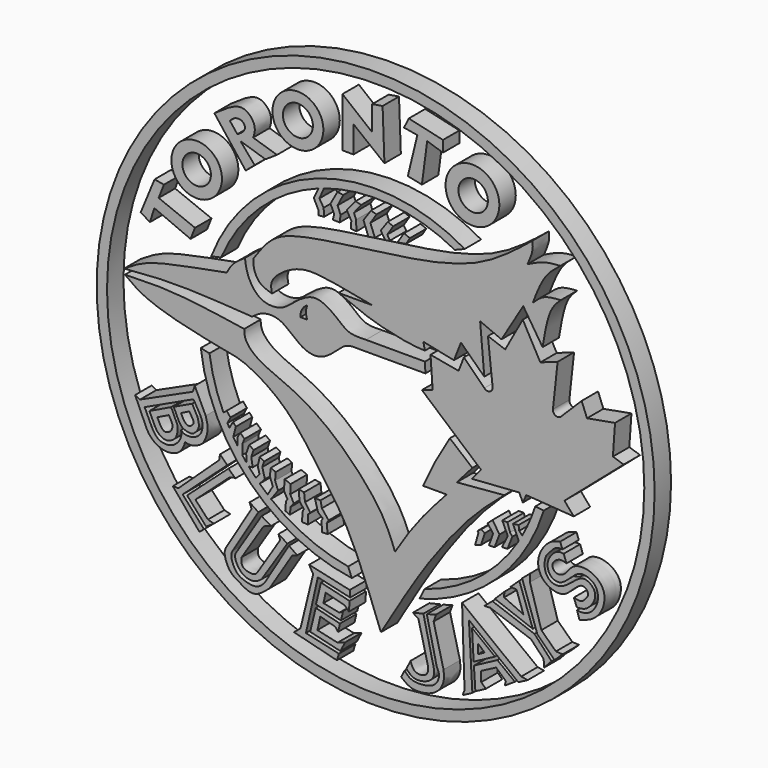
from build123d import *

# Parameters (mm, degrees)
F0_R     = 86.3413531424
F0_R_2   = 83.1380480695
F1_DEPTH = 6.35
F0_R_3   = 7.8789103403
F0_R_4   = 4.6380734479
F0_R_5   = 8.3244064096
F0_R_6   = 4.5488464078
F0_R_7   = 7.8253393062
F0_R_8   = 4.4151925566


with BuildPart() as f1:
    # F0 (on Front) → F1 (new body)
    with BuildSketch(Plane.XZ):
        with Locations((103.031180799, 95.9219709039)):
            Circle(F0_R)
        with Locations((103.031180799, 95.9219709039)):
            Circle(F0_R_2, mode=Mode.SUBTRACT)
    extrude(amount=F1_DEPTH)


with BuildPart() as f1b:
    # F0 (on Front) → F1, piece 2 (new body)
    with BuildSketch(Plane.XZ):
        with BuildLine():
            ThreePointArc((147.3083680993, 68.8155244448), (134.8042261554, 54.8646652976), (118.1625116195, 46.2604004246))
            Line((118.1625116195, 46.2604004246), (116.5973385643, 43.1300521934))
            ThreePointArc((116.5973385643, 43.1300521934), (140.56012864, 56.3921670644), (155.0479381108, 79.6344211676))
            Line((155.0479381108, 79.6344211676), (152.4171286424, 79.9139444647))
            ThreePointArc((152.4171286424, 79.9139444647), (150.6252567937, 75.1847414583), (148.3817446246, 70.6523227945))
            ThreePointArc((148.3817446246, 70.6523227945), (147.8544660424, 69.7284248505), (147.3083680993, 68.8155244448))
        make_face()
        with BuildLine():
            Line((145.5425322056, 72.9509443045), (147.3083680993, 68.8155244448))
            ThreePointArc((147.3083680993, 68.8155244448), (147.8544660424, 69.7284248505), (148.3817446246, 70.6523227945))
            Line((148.3817446246, 70.6523227945), (147.4613398314, 71.6612488031))
            Line((147.4613398314, 71.6612488031), (147.2726166248, 73.1711387634))
            Line((147.2726166248, 73.1711387634), (145.5425322056, 72.9509443045))
        make_face()
    extrude(amount=F1_DEPTH)


with BuildPart() as f1c:
    # F0 (on Front) → F1, piece 3 (new body)
    with BuildSketch(Plane.XZ):
        with BuildLine():
            Line((51.6026031998, 88.8275955975), (48.9147157589, 89.4077150596))
            ThreePointArc((48.9147157589, 89.4077150596), (64.1807826745, 57.6901270664), (95.6492936354, 41.9170168761))
            Line((95.6492936354, 41.9170168761), (94.5090451372, 44.7106249088))
            ThreePointArc((94.5090451372, 44.7106249088), (81.9000965732, 48.501447559), (70.6502899912, 55.3423372762))
            ThreePointArc((70.6502899912, 55.3423372762), (70.115809711, 55.7746534218), (69.5871006289, 56.2140087749))
            ThreePointArc((69.5871006289, 56.2140087749), (68.3513199524, 57.2886173538), (67.1500481163, 58.4016687693))
            ThreePointArc((67.1500481163, 58.4016687693), (66.5511264504, 58.983719868), (65.9616453548, 59.5753301125))
            ThreePointArc((65.9616453548, 59.5753301125), (64.8429965328, 60.752504924), (63.7617125025, 61.9640908968))
            ThreePointArc((63.7617125025, 61.9640908968), (63.43044974, 62.350988576), (63.1029986811, 62.7411175751))
            ThreePointArc((63.1029986811, 62.7411175751), (62.4252381027, 63.5740780419), (61.7648512125, 64.4208789018))
            ThreePointArc((61.7648512125, 64.4208789018), (61.0137454914, 65.429941043), (60.2873081661, 66.4569050257))
            ThreePointArc((60.2873081661, 66.4569050257), (59.6233759404, 67.4440631116), (58.9822375149, 68.4461751843))
            ThreePointArc((58.9822375149, 68.4461751843), (58.3639510652, 69.4631851651), (57.7691413004, 70.4941016402))
            ThreePointArc((57.7691413004, 70.4941016402), (57.4587222425, 71.0547278725), (57.155246887, 71.6191430321))
            ThreePointArc((57.155246887, 71.6191430321), (56.5262459763, 72.8455805448), (55.9300250893, 74.0882839575))
            ThreePointArc((55.9300250893, 74.0882839575), (53.2181412071, 81.296997691), (51.6026031998, 88.8275955975))
        make_face()
        with BuildLine():
            Line((56.9120161235, 74.9070867896), (55.9300250893, 74.0882839575))
            ThreePointArc((55.9300250893, 74.0882839575), (56.5262459763, 72.8455805448), (57.155246887, 71.6191430321))
            Line((57.155246887, 71.6191430321), (58.1148564816, 73.4815001488))
            Line((58.1148564816, 73.4815001488), (56.9120161235, 74.9070867896))
        make_face()
        with BuildLine():
            Line((58.8709115982, 72.4884793162), (57.7691413004, 70.4941016402))
            ThreePointArc((57.7691413004, 70.4941016402), (58.3639510652, 69.4631851651), (58.9822375149, 68.4461751843))
            Line((58.9822375149, 68.4461751843), (59.7831308842, 71.5290755033))
            Line((59.7831308842, 71.5290755033), (58.8709115982, 72.4884793162))
        make_face()
        with BuildLine():
            Line((60.2873081661, 68.8241523461), (60.2873081661, 66.4569050257))
            ThreePointArc((60.2873081661, 66.4569050257), (61.0137454914, 65.429941043), (61.7648512125, 64.4208789018))
            Line((61.7648512125, 64.4208789018), (61.7648512125, 67.4240812659))
            Line((61.7648512125, 67.4240812659), (62.4568797648, 69.0440535545))
            Line((62.4568797648, 69.0440535545), (61.1357353628, 70.2865645289))
            Line((61.1357353628, 70.2865645289), (60.2873081661, 68.8241523461))
        make_face()
        with BuildLine():
            ThreePointArc((63.1029986811, 62.7411175751), (63.43044974, 62.350988576), (63.7617125025, 61.9640908968))
            Line((63.7617125025, 61.9640908968), (65.0048106909, 62.123760581))
            Line((65.0048106909, 62.123760581), (64.5329728723, 64.7660568357))
            Line((64.5329728723, 64.7660568357), (65.2721822262, 66.920787096))
            Line((65.2721822262, 66.920787096), (63.9195814729, 67.9273754358))
            Line((63.9195814729, 67.9273754358), (62.96017766, 65.2536228299))
            Line((62.96017766, 65.2536228299), (63.1029986811, 62.7411175751))
        make_face()
        with BuildLine():
            ThreePointArc((65.9616453548, 59.5753301125), (66.5511264504, 58.983719868), (67.1500481163, 58.4016687693))
            Line((67.1500481163, 58.4016687693), (68.748511374, 60.1065568626))
            Line((68.748511374, 60.1065568626), (67.9659470916, 63.1837621331))
            Line((67.9659470916, 63.1837621331), (68.4965029359, 64.8682713509))
            Line((68.4965029359, 64.8682713509), (67.1833828092, 65.7171532512))
            Line((67.1833828092, 65.7171532512), (66.5334537625, 63.0643889308))
            Line((66.5334537625, 63.0643889308), (67.0905336738, 60.9023831785))
            Line((67.0905336738, 60.9023831785), (65.9616453548, 59.5753301125))
        make_face()
        with BuildLine():
            ThreePointArc((69.5871006289, 56.2140087749), (70.115809711, 55.7746534218), (70.6502899912, 55.3423372762))
            Line((70.6502899912, 55.3423372762), (72.8397592902, 58.3484321833))
            Line((72.8397592902, 58.3484321833), (71.9113647938, 60.7402287424))
            Line((71.9113647938, 60.7402287424), (72.1001923084, 63.1477609277))
            Line((72.1001923084, 63.1477609277), (70.5895796418, 63.8243928552))
            Line((70.5895796418, 63.8243928552), (70.2748671174, 61.4325925708))
            Line((70.2748671174, 61.4325925708), (71.2347403169, 58.9463822544))
            Line((71.2347403169, 58.9463822544), (69.5871006289, 56.2140087749))
        make_face()
    extrude(amount=F1_DEPTH)


with BuildPart() as f1d:
    # F0 (on Front) → F1, piece 4 (new body)
    with BuildSketch(Plane.XZ):
        with BuildLine():
            ThreePointArc((130.5909766711, 142.9483993153), (84.998217789, 147.3596959967), (52.1404570115, 115.4453299904))
            Line((52.1404570115, 115.4453299904), (55.2052152042, 116.1186481005))
            ThreePointArc((55.2052152042, 116.1186481005), (67.2921720529, 133.5776744388), (85.3582697834, 144.7368966039))
            ThreePointArc((85.3582697834, 144.7368966039), (86.1877646377, 145.0292828532), (87.0220936823, 145.3075749253))
            ThreePointArc((87.0220936823, 145.3075749253), (107.6444471834, 147.632187768), (127.5296217117, 141.6937432938))
            Line((127.5296217117, 141.6937432938), (130.5909766711, 142.9483993153))
        make_face()
        with BuildLine():
            ThreePointArc((87.0220936823, 145.3075749253), (86.1877646377, 145.0292828532), (85.3582697834, 144.7368966039))
            Line((85.3582697834, 144.7368966039), (83.8721096516, 141.6685283184))
            Line((83.8721096516, 141.6685283184), (85.278019309, 138.902798295))
            Line((85.278019309, 138.902798295), (85.278019309, 137.4046951532))
            Line((85.278019309, 137.4046951532), (87.0757475495, 137.5429779291))
            Line((87.0757475495, 137.5429779291), (86.9374573231, 139.986038208))
            Line((86.9374573231, 139.986038208), (85.6237336993, 142.1064287424))
            Line((85.6237336993, 142.1064287424), (87.0220936823, 145.3075749253))
        make_face()
    extrude(amount=F1_DEPTH)


with BuildPart() as f1e:
    # F0 (on Front) → F1, piece 5 (new body)
    with BuildSketch(Plane.XZ):
        with BuildLine():
            add(Edge.make_bspline(
                [(65.1605650783, 119.0443858504), (66.8778376252, 121.5129392999), (70.4109060542, 126.5916720109), (79.9235957481, 130.7139890188), (110.1374116444, 133.9828883244), (135.222430189, 138.8339439937), (146.3601247065, 147.8218221424), (151.5567153692, 152.0153582096)],
                knots=[0, 0, 0, 0, 0.1391278046, 0.2862376476, 0.5460671762, 0.7882054433, 1, 1, 1, 1], degree=3))
            add(Edge.make_bspline(
                [(65.1605650783, 119.0443858504), (65.1761761693, 118.1416763553), (65.2095890258, 116.209581882), (66.9509015853, 112.6183397292), (69.5998832246, 111.8216078708), (70.9610208869, 111.4122197032)],
                knots=[0, 0, 0, 0, 0.2989041205, 0.63975288, 1, 1, 1, 1], degree=3))
            add(Edge.make_bspline(
                [(70.9610208869, 111.4122197032), (70.7064543789, 112.6000383971), (70.0542774567, 115.6431250383), (78.5588548833, 121.5103784794), (86.7278880375, 121.319656762), (96.3330449421, 119.4304990241), (101.8915474415, 118.3372437954)],
                knots=[0, 0, 0, 0, 0.1632480059, 0.4182269808, 0.6633280629, 1, 1, 1, 1], degree=3))
            add(Edge.make_bspline(
                [(91.5042832494, 118.2865723968), (94.9667046467, 118.303462863), (98.4291260441, 118.3203533292), (101.8915474415, 118.3372437954)],
                knots=[0, 0, 0, 0, 10.3873877846, 10.3873877846, 10.3873877846, 10.3873877846], degree=3))
            add(Edge.make_bspline(
                [(91.5042832494, 118.2865723968), (95.4103000455, 116.6689675882), (102.9409801099, 113.550275345), (114.0365493527, 111.4182928611), (117.1070508324, 111.2911466343), (118.2578355074, 111.243493855)],
                knots=[0, 0, 0, 0, 0.4025367258, 0.7760784079, 1, 1, 1, 1], degree=3))
            Line((118.2578355074, 111.243493855), (117.8089082241, 113.522939384))
            Line((117.8089082241, 113.522939384), (127.2610574961, 111.5468814969))
            Line((127.2610574961, 111.5468814969), (129.4347345829, 117.079846561))
            Line((129.4347345829, 117.079846561), (136.6473585367, 110.1306974888))
            Line((136.6473585367, 110.1306974888), (135.3629082441, 124.8194202781))
            Line((135.3629082441, 124.8194202781), (141.9620066881, 122.0207512379))
            Line((141.9620066881, 122.0207512379), (148.6962139606, 133.2910507917))
            Line((148.6962139606, 133.2910507917), (154.6910554171, 124.0390092134))
            add(Edge.make_bspline(
                [(160.315155983, 138.6734396219), (159.2455875755, 137.6606965238), (156.5295767546, 135.0889851736), (155.384935522, 128.2094032809), (154.6910554171, 124.0390092134)],
                knots=[0, 0, 0, 0, 0.393801232, 1, 1, 1, 1], degree=3))
            add(Edge.make_bspline(
                [(151.6671776772, 135.1648271084), (152.7209926622, 136.1815330098), (154.935600551, 138.3181556068), (158.4651387096, 138.551258231), (160.315155983, 138.6734396219)],
                knots=[0, 0, 0, 0, 0.4758472099, 1, 1, 1, 1], degree=3))
            add(Edge.make_bspline(
                [(160.1669043303, 147.9638516903), (158.5547438369, 146.6889334698), (154.9894110066, 143.8694202723), (152.843020417, 138.2456560751), (151.6671776772, 135.1648271084)],
                knots=[0, 0, 0, 0, 0.4521767168, 1, 1, 1, 1], degree=3))
            add(Edge.make_bspline(
                [(150.0364094973, 145.1470702887), (151.760692317, 145.9999334812), (155.1077875128, 147.6554706482), (158.5149626664, 147.8631567449), (160.1669043303, 147.9638516903)],
                knots=[0, 0, 0, 0, 0.5151579859, 1, 1, 1, 1], degree=3))
            add(Edge.make_bspline(
                [(151.5567153692, 152.0153582096), (151.6401552323, 151.1871213753), (151.8331461293, 149.2714642344), (150.6870113993, 146.6405215258), (150.0364094973, 145.1470702887)],
                knots=[0, 0, 0, 0, 0.432351289, 1, 1, 1, 1], degree=3))
        make_face()
    extrude(amount=F1_DEPTH)


with BuildPart() as f1f:
    # F0 (on Front) → F1, piece 6 (new body)
    with BuildSketch(Plane.XZ):
        with BuildLine():
            add(Edge.make_bspline(
                [(25.1967553049, 103.3449247479), (27.3040968371, 104.7393627023), (32.4641344694, 108.1537842428), (50.5762950972, 111.2823313326), (55.2229375422, 112.2109965294), (56.9541603327, 112.5569939613)],
                knots=[0, 0, 0, 0, 0.3022241239, 0.7400261557, 1, 1, 1, 1], degree=3))
            add(Edge.make_bspline(
                [(25.1967553049, 103.3449247479), (29.9715334206, 103.7590919436), (40.7871203818, 104.6972426205), (56.1858731237, 103.685420688), (64.7865086794, 103.1202897429)],
                knots=[0, 0, 0, 0, 0.4414719361, 1, 1, 1, 1], degree=3))
            add(Edge.make_bspline(
                [(64.7865086794, 103.1202897429), (65.8668973717, 103.9080368704), (68.1814863805, 105.5956802675), (74.1229212632, 105.629850452), (79.4777048259, 99.5938625168), (85.4832150354, 98.1867823774), (90.0852174163, 101.3548826723), (93.694568367, 105.2928580339), (98.082420715, 105.0210518449), (99.9919539194, 105.0507986742), (100.8540317416, 105.0642281771)],
                knots=[0, 0, 0, 0, 0.1136037838, 0.2433809899, 0.4013829827, 0.5347427751, 0.6644027588, 0.7926653345, 0.9063966961, 1, 1, 1, 1], degree=3))
            Line((100.8540317416, 105.0642281771), (118.4250637889, 105.0808951259))
            Line((118.4250637889, 105.0808951259), (118.2891801, 108.2712113857))
            Line((118.2891801, 108.2712113857), (100.034929812, 108.2712113857))
            add(Edge.make_bspline(
                [(62.5645443797, 118.3710470796), (62.7810828536, 116.8203199403), (63.2439830099, 113.5052885639), (67.1459023608, 107.817655531), (73.9886371488, 107.8306557792), (77.4019191042, 111.1699255534), (81.1499566889, 113.7985632868), (85.4234713853, 115.2807346354), (91.3316282439, 111.2904547181), (94.4912731866, 108.103824159), (98.1342859466, 108.2138226391), (100.034929812, 108.2712113857)],
                knots=[0, 0, 0, 0, 0.1079264135, 0.2307172152, 0.3501145928, 0.455522384, 0.5593277087, 0.6585426343, 0.7849741393, 0.887816044, 1, 1, 1, 1], degree=3))
            add(Edge.make_bspline(
                [(62.5645443797, 118.3710470796), (62.1619489758, 118.1183126282), (61.1729889871, 117.4974802547), (58.4413848848, 115.3726745542), (57.4458065929, 113.4878008334), (56.9541603327, 112.5569939613)],
                knots=[0, 0, 0, 0, 0.2579038412, 0.6335307789, 1, 1, 1, 1], degree=3))
        make_face()
        with BuildLine():
            ThreePointArc((79.7450765967, 107.8225299716), (80.2463337926, 110.1185380343), (81.8977057934, 111.7906272411))
            ThreePointArc((81.8977057934, 111.7906272411), (81.4659620101, 109.8248859653), (81.8458348513, 107.8484654427))
            Line((81.8458348513, 107.8484654427), (79.7450765967, 107.8225299716))
        make_face(mode=Mode.SUBTRACT)
    extrude(amount=F1_DEPTH)


with BuildPart() as f1g:
    # F0 (on Front) → F1, piece 7 (new body)
    with BuildSketch(Plane.XZ):
        with BuildLine():
            Line((153.9957672358, 119.6609884501), (148.5578864813, 129.5398026705))
            Line((148.5578864813, 129.5398026705), (143.1200057268, 119.6609884501))
            Line((143.1200057268, 119.6609884501), (137.7727538347, 121.5642467141))
            Line((137.7727538347, 121.5642467141), (139.2228603363, 108.1508100033))
            ThreePointArc((139.2228603363, 108.1508100033), (138.3571175254, 106.656984618), (136.6722881794, 107.0343106985))
            Line((136.6722881794, 107.0343106985), (130.3365975618, 113.3399754763))
            Line((130.3365975618, 113.3399754763), (128.6851167679, 109.1362014413))
            Line((128.6851167679, 109.1362014413), (120.0073137879, 110.6976047158))
            Line((120.0073137879, 110.6976047158), (120.6679046154, 101.2991517782))
            Line((120.6679046154, 101.2991517782), (117.3349097371, 100.2181842923))
            Line((117.3349097371, 100.2181842923), (135.6661170721, 84.4167545438))
            Line((135.6661170721, 84.4167545438), (132.773819657, 81.0614060446))
            Line((132.773819657, 81.0614060446), (147.4750339985, 82.0971429348))
            Line((147.4750339985, 82.0971429348), (148.5578864813, 79.6925723553))
            Line((148.5578864813, 79.6925723553), (149.6407389641, 82.0971429348))
            Line((149.6407389641, 82.0971429348), (164.3419533056, 81.0614060446))
            Line((164.3419533056, 81.0614060446), (161.4496558905, 84.4167545438))
            Line((161.4496558905, 84.4167545438), (179.7808632255, 100.2181842923))
            Line((179.7808632255, 100.2181842923), (176.4478683472, 101.2991517782))
            Line((176.4478683472, 101.2991517782), (177.1084591746, 110.6976047158))
            Line((177.1084591746, 110.6976047158), (168.4306561947, 109.1362014413))
            Line((168.4306561947, 109.1362014413), (166.7791754007, 113.3399754763))
            Line((166.7791754007, 113.3399754763), (160.4434847832, 107.0343106985))
            ThreePointArc((160.4434847832, 107.0343106985), (158.7586554371, 106.656984618), (157.8929126263, 108.1508100033))
            Line((157.8929126263, 108.1508100033), (159.3430191278, 121.5642467141))
            Line((159.3430191278, 121.5642467141), (153.9957672358, 119.6609884501))
        make_face()
    extrude(amount=F1_DEPTH)


with BuildPart() as f1h:
    # F0 (on Front) → F1, piece 8 (new body)
    with BuildSketch(Plane.XZ):
        with BuildLine():
            add(Edge.make_bspline(
                [(25.4391785711, 101.7691716552), (30.0819421715, 101.9373475003), (40.4646043806, 102.313440953), (54.5665174618, 100.1663488978), (62.3625479639, 98.9793613553)],
                knots=[0, 0, 0, 0, 0.4471650437, 1, 1, 1, 1], degree=3))
            add(Edge.make_bspline(
                [(25.4391785711, 101.7691716552), (27.4951677939, 100.2010333845), (32.6963862517, 96.2339747892), (53.7919926338, 91.5360298149), (62.6667020346, 90.4660345952), (76.1675062641, 81.8773948587), (85.1809430093, 68.5570252624), (94.9490355887, 55.8282536231), (101.1341707007, 39.4515366233), (104.6594902873, 30.1173571497)],
                knots=[0, 0, 0, 0, 0.1078526072, 0.2728443151, 0.3840716275, 0.52293785, 0.667189915, 0.8103094128, 1, 1, 1, 1], degree=3))
            add(Edge.make_bspline(
                [(142.8586542606, 79.8605903983), (139.8099959288, 77.2901032161), (132.7752691758, 71.3587481803), (118.9267540138, 54.1605827862), (109.6282733945, 38.4907618667), (104.6594902873, 30.1173571497)],
                knots=[0, 0, 0, 0, 0.2626080184, 0.6059634932, 1, 1, 1, 1], degree=3))
            Line((142.8586542606, 79.8605903983), (128.1391531229, 78.5893574357))
            Line((128.1391531229, 78.5893574357), (132.9556107521, 84.0778797865))
            Line((132.9556107521, 84.0778797865), (125.9915083647, 89.889511466))
            add(Edge.make_bspline(
                [(125.9915083647, 89.889511466), (124.1906776032, 86.884529911), (120.831371918, 81.2789772755), (118.6989388734, 76.4671217587), (117.7096441388, 74.2347687483)],
                knots=[0, 0, 0, 0, 0.5360723109, 1, 1, 1, 1], degree=3))
            Line((117.7096441388, 74.2347687483), (124.9815225601, 74.2347687483))
            add(Edge.make_bspline(
                [(109.0237796307, 53.4291043878), (111.0607083235, 56.6835559182), (115.3540422303, 63.5431220642), (121.6648260608, 70.5514636763), (124.9815225601, 74.2347687483)],
                knots=[0, 0, 0, 0, 0.4744398496, 1, 1, 1, 1], degree=3))
            add(Edge.make_bspline(
                [(62.3625479639, 98.9793613553), (62.3939304569, 98.0520448539), (62.470120325, 95.8007220626), (67.1036326561, 91.1212871301), (79.0408742875, 87.1555023958), (92.4624754667, 77.7456992381), (105.2124808885, 63.5789766808), (107.8826662406, 56.468004239), (109.0237796307, 53.4291043878)],
                knots=[0, 0, 0, 0, 0.0876826859, 0.212874492, 0.3948990845, 0.6080658661, 0.8325055271, 1, 1, 1, 1], degree=3))
        make_face()
    extrude(amount=F1_DEPTH)


with BuildPart() as f1i:
    # F0 (on Front) → F1, piece 9 (new body)
    with BuildSketch(Plane.XZ):
        Polygon((45.7493290305, 118.0791184306), (47.1274256706, 121.5687170625), (35.8816534281, 126.0549873114), (37.5066287816, 130.2057057619), (34.6122793853, 130.7036727667), (30.3303021938, 120.3440725803), (33.1689864397, 118.5628324747), (34.5361232758, 122.8588074446), align=None)
    extrude(amount=F1_DEPTH)


with BuildPart() as f1j:
    # F0 (on Front) → F1, piece 10 (new body)
    with BuildSketch(Plane.XZ):
        with BuildLine():
            add(Edge.make_bspline(
                [(53.1252250075, 154.7500044107), (55.2469486953, 156.2413880414), (58.8098820474, 158.7458142818), (62.4338563704, 159.3498216887), (65.3452902263, 156.7860195347), (65.8141525821, 153.9353043584), (65.3288470884, 152.6082080035), (65.105214715, 151.9966721535)],
                knots=[0, 0, 0, 0, 0.283267468, 0.4756807474, 0.6736240285, 0.84960353, 1, 1, 1, 1], degree=3))
            Line((53.1252250075, 154.7500044107), (62.8135204315, 142.2608792782))
            Line((62.8135204315, 142.2608792782), (65.5893757939, 144.6471214294))
            Line((65.5893757939, 144.6471214294), (61.1652935744, 149.7935447907))
            Line((61.1652935744, 149.7935447907), (68.9228177071, 147.3327279091))
            Line((68.9228177071, 147.3327279091), (72.4971592426, 149.693518877))
            Line((72.4971592426, 149.693518877), (65.105214715, 151.9966721535))
        make_face()
        with BuildLine():
            Line((60.2364838123, 151.348516345), (57.8906238079, 154.3007344007))
            add(Edge.make_bspline(
                [(57.8906238079, 154.3007344007), (58.4380867229, 154.7951363586), (59.5217921733, 155.7738073915), (61.9341600232, 155.7245852448), (62.9476560436, 153.6651432613), (61.6809151257, 152.170733141), (60.7159422125, 151.6214394989), (60.2364838123, 151.348516345)],
                knots=[0, 0, 0, 0, 0.2140840398, 0.4237803775, 0.6200878393, 0.8112360728, 1, 1, 1, 1], degree=3))
        make_face(mode=Mode.SUBTRACT)
    extrude(amount=F1_DEPTH)


with BuildPart() as f1k:
    # F0 (on Front) → F1, piece 11 (new body)
    with BuildSketch(Plane.XZ):
        with Locations((78.9697542787, 161.17811203)):
            Circle(F0_R_3)
        with Locations((78.9697542787, 161.17811203)):
            Circle(F0_R_4, mode=Mode.SUBTRACT)
    extrude(amount=F1_DEPTH)


with BuildPart() as f1l:
    # F0 (on Front) → F1, piece 12 (new body)
    with BuildSketch(Plane.XZ):
        Polygon((105.7477369905, 158.2026481628), (105.1767095923, 173.6358851194), (101.9640862942, 173.1107831001), (101.9640862942, 165.42981565), (92.7540138364, 172.8455275297), (92.7540138364, 157.5022041798), (96.1784869432, 157.5022041798), (96.1784869432, 165.7617539167), align=None)
    extrude(amount=F1_DEPTH)


with BuildPart() as f1m:
    # F0 (on Front) → F1, piece 13 (new body)
    with BuildSketch(Plane.XZ):
        Polygon((112.9893511534, 157.0811718702), (117.3376590014, 156.1619192362), (118.9757287502, 168.5630083084), (123.8637119532, 166.9919341803), (123.8637119532, 170.4729348421), (113.2804900408, 172.8813052177), (111.8034347892, 169.9022501707), (115.9320175648, 169.1992431879), align=None)
    extrude(amount=F1_DEPTH)


with BuildPart() as f1n:
    # F0 (on Front) → F1, piece 14 (new body)
    with BuildSketch(Plane.XZ):
        with Locations((132.9881995916, 158.4182977676)):
            Circle(F0_R_5)
        with Locations((133.2059800625, 158.3469808102)):
            Circle(F0_R_6, mode=Mode.SUBTRACT)
    extrude(amount=F1_DEPTH)


with BuildPart() as f1o:
    # F0 (on Front) → F1, piece 15 (new body)
    with BuildSketch(Plane.XZ):
        with BuildLine():
            Line((30.084611848, 69.2335367203), (28.5908672959, 69.9970424175))
            Line((28.5908672959, 69.9970424175), (32.2739779949, 61.7518611252))
            add(Edge.make_bspline(
                [(32.2739779949, 61.7518611252), (32.7749833614, 60.9635409459), (33.8725362138, 59.2365673057), (37.7843402929, 57.3661795763), (40.9000261821, 58.0772316706), (42.4748576233, 58.8884277898), (43.7190339293, 60.8511833229), (43.92516752, 61.788340814), (44.0159887075, 62.2012466192)],
                knots=[0, 0, 0, 0, 0.1805400151, 0.3955091539, 0.5798726097, 0.7192386574, 0.8762982857, 1, 1, 1, 1], degree=3))
            add(Edge.make_bspline(
                [(50.4372827709, 71.4342072606), (50.768796352, 70.2681071733), (51.4423387053, 67.8989197804), (50.0208490553, 63.9368372151), (48.3439726978, 62.6064898882), (45.6286973181, 61.7319686813), (44.5064816628, 62.0585193335), (44.0159887075, 62.2012466192)],
                knots=[0, 0, 0, 0, 0.2317101951, 0.4707699442, 0.6474136486, 0.8458931484, 1, 1, 1, 1], degree=3))
            Line((50.4372827709, 71.4342072606), (47.0445714891, 78.5238817334))
            Line((47.0445714891, 78.5238817334), (46.4649833739, 76.70263201))
            Line((46.4649833739, 76.70263201), (30.084611848, 69.2335367203))
        make_face()
        with BuildLine():
            Line((33.7571738878, 62.9248380445), (31.5462499857, 67.6518827677))
            Line((31.5462499857, 67.6518827677), (46.6555319726, 74.7187659144))
            Line((46.6555319726, 74.7187659144), (48.8234609365, 70.9855034947))
            add(Edge.make_bspline(
                [(48.8234609365, 70.9855034947), (49.0819708256, 70.3935862537), (49.6586394805, 69.0731720892), (49.237163999, 65.7047735608), (46.3921689965, 63.9972381576), (43.6765691296, 64.193013021), (43.0678826774, 64.8492305233), (42.8228862584, 65.1133581996)],
                knots=[0, 0, 0, 0, 0.1877571763, 0.4188376649, 0.6505028982, 0.8593273465, 1, 1, 1, 1], degree=3))
            add(Edge.make_bspline(
                [(42.8228862584, 65.1133581996), (42.8995880194, 64.5288190639), (43.0701928475, 63.2286507568), (41.5554270585, 60.7324634798), (38.9094693245, 59.408386698), (35.4556323147, 59.9614920092), (34.3283304255, 61.9283258929), (33.7571738878, 62.9248380445)],
                knots=[0, 0, 0, 0, 0.1629627988, 0.3624719943, 0.5673253374, 0.7807819142, 1, 1, 1, 1], degree=3))
        make_face(mode=Mode.SUBTRACT)
    extrude(amount=F1_DEPTH)


with BuildPart() as f1p:
    # F0 (on Front) → F1, piece 16 (new body)
    with BuildSketch(Plane.XZ):
        with BuildLine():
            Line((33.0113917589, 67.0752748847), (34.7925238311, 63.375480473))
            add(Edge.make_bspline(
                [(34.7925238311, 63.375480473), (35.0775184998, 62.8565718788), (35.6921398313, 61.7374902743), (38.0879074589, 60.4498929431), (40.1144582874, 61.3870935102), (41.5870528741, 62.6273809347), (41.9177078829, 65.8310003744), (41.5595239996, 66.4209627993), (41.4349101484, 66.626213491)],
                knots=[0, 0, 0, 0, 0.1617435236, 0.348817121, 0.5186377126, 0.6833715959, 0.8898434947, 1, 1, 1, 1], degree=3))
            Line((41.4349101484, 66.626213491), (39.7495812228, 70.3191322528))
            Line((39.7495812228, 70.3191322528), (33.0113917589, 67.0752748847))
        make_face()
        with BuildLine():
            add(Edge.make_bspline(
                [(39.0181578696, 67.9107233882), (39.3521406209, 67.3612992199), (39.9734686595, 66.3391726595), (40.3585117661, 64.9323679736), (39.4065180237, 63.2149036456), (37.5045449143, 62.7910345829), (36.4835226493, 64.0908443815), (35.8268386909, 65.4262056166), (35.4576520622, 66.176943481)],
                knots=[0, 0, 0, 0, 0.1723413883, 0.320616967, 0.4896060074, 0.6516265134, 0.8041450056, 1, 1, 1, 1], degree=3))
            Line((35.4576520622, 66.176943481), (39.0181578696, 67.9107233882))
        make_face(mode=Mode.SUBTRACT)
    extrude(amount=F1_DEPTH)


with BuildPart() as f1q:
    # F0 (on Front) → F1, piece 17 (new body)
    with BuildSketch(Plane.XZ):
        with BuildLine():
            Line((40.5272841454, 70.6554576755), (42.1947091818, 67.1063810587))
            add(Edge.make_bspline(
                [(42.1947091818, 67.1063810587), (42.5300203172, 66.6059812645), (43.2534498254, 65.5263750754), (45.9643010197, 64.9343952109), (47.0261507091, 65.6262016891), (48.7203927869, 67.4674823606), (48.1852515678, 69.3114875856), (47.9004643857, 70.2928155661)],
                knots=[0, 0, 0, 0, 0.1892913736, 0.4083937301, 0.5618475325, 0.7668275175, 1, 1, 1, 1], degree=3))
            Line((47.9004643857, 70.2928155661), (46.2758727372, 73.3677372336))
            Line((46.2758727372, 73.3677372336), (40.5272841454, 70.6554576755))
        make_face()
        with BuildLine():
            add(Edge.make_bspline(
                [(42.7959747612, 69.7186216712), (43.047642654, 69.1511576598), (43.5409352666, 68.0388751126), (44.9829181822, 66.4963706403), (46.8393950574, 67.849105025), (46.5990822652, 69.119399867), (45.7980453979, 70.2741922494), (45.3262329102, 70.9543675184)],
                knots=[0, 0, 0, 0, 0.2093713151, 0.4103873638, 0.6113362611, 0.7710761976, 1, 1, 1, 1], degree=3))
            Line((42.7959747612, 69.7186216712), (45.3262329102, 70.9543675184))
        make_face(mode=Mode.SUBTRACT)
    extrude(amount=F1_DEPTH)


with BuildPart() as f1r:
    # F0 (on Front) → F1, piece 18 (new body)
    with BuildSketch(Plane.XZ):
        Polygon((42.0019701123, 48.9689558744), (40.2475222945, 48.9689558744), (48.4948754311, 39.1794070601), (49.9138982921, 40.3748842845), (43.3076843619, 47.6965904236), (57.1298776725, 60.1680505258), (54.8735894263, 62.4050199986), (54.5935668051, 60.7121512294), align=None)
    extrude(amount=F1_DEPTH)


with BuildPart() as f1s:
    # F0 (on Front) → F1, piece 19 (new body)
    with BuildSketch(Plane.XZ):
        Polygon((59.1355338693, 57.3903694749), (59.5765225589, 57.3363490403), (57.5092588319, 59.385912458), (44.6798056364, 47.8761643171), (50.5935712321, 41.2843277287), (52.980992943, 42.9032854736), (51.1294156313, 43.4014163911), (47.2444631159, 47.572825104), (57.8899629671, 57.1232728319), align=None)
    extrude(amount=F1_DEPTH)


with BuildPart() as f1t:
    # F0 (on Front) → F1, piece 20 (new body)
    with BuildSketch(Plane.XZ):
        with BuildLine():
            Line((66.7242109776, 50.4824742675), (64.0202015638, 52.2900372744))
            Line((64.0202015638, 52.2900372744), (64.6236911416, 50.680808723))
            Line((64.6236911416, 50.680808723), (56.8242445588, 37.761926651))
            add(Edge.make_bspline(
                [(56.8242445588, 37.761926651), (56.5676145385, 37.2745883782), (55.9068287024, 36.0197615746), (57.5079599547, 31.3390733944), (60.8664515095, 29.4597501756), (65.4071147291, 26.6832553249), (68.507722817, 29.3797027929), (70.1521411538, 30.8097731322)],
                knots=[0, 0, 0, 0, 0.1342385427, 0.3456451728, 0.5458891784, 0.7591607385, 1, 1, 1, 1], degree=3))
            Line((70.1521411538, 30.8097731322), (77.2129967809, 42.0901700854))
            Line((77.2129967809, 42.0901700854), (78.7653923035, 42.636051774))
            Line((78.7653923035, 42.636051774), (76.2063041329, 44.4313026965))
            Line((76.2063041329, 44.4313026965), (68.6753094196, 31.8774543703))
            add(Edge.make_bspline(
                [(58.728441596, 37.323653698), (58.5230264271, 36.8687220199), (57.9958517355, 35.701191558), (59.6709627467, 31.6246690145), (62.6263598052, 30.2447432329), (66.4668279016, 29.5192915207), (67.9592674068, 31.1128821247), (68.6753094196, 31.8774543703)],
                knots=[0, 0, 0, 0, 0.1465737445, 0.3761648615, 0.5851241919, 0.8009510552, 1, 1, 1, 1], degree=3))
            Line((58.728441596, 37.323653698), (66.7242109776, 50.4824742675))
        make_face()
    extrude(amount=F1_DEPTH)


with BuildPart() as f1u:
    # F0 (on Front) → F1, piece 21 (new body)
    with BuildSketch(Plane.XZ):
        with BuildLine():
            Line((68.358771503, 47.1663214266), (70.66360116, 47.9982383549))
            Line((70.66360116, 47.9982383549), (67.7331537008, 49.7590638697))
            Line((67.7331537008, 49.7590638697), (59.5980621874, 36.8272326887))
            add(Edge.make_bspline(
                [(59.5980621874, 36.8272326887), (59.55062306, 36.4261853148), (59.438542995, 35.478667555), (60.5401445667, 33.2608556021), (62.4429161253, 31.3158868178), (65.6771009548, 30.977799307), (67.0440481349, 32.0071660769), (67.6952302456, 32.4975326657)],
                knots=[0, 0, 0, 0, 0.1489567751, 0.351926478, 0.5681800933, 0.7942909555, 1, 1, 1, 1], degree=3))
            Line((67.6952302456, 32.4975326657), (75.7021382451, 44.8366180062))
            Line((75.7021382451, 44.8366180062), (72.953954339, 46.5528592467))
            Line((72.953954339, 46.5528592467), (73.4739005566, 45.0526252389))
            Line((73.4739005566, 45.0526252389), (66.4487108588, 33.993948251))
            add(Edge.make_bspline(
                [(66.4487108588, 33.993948251), (66.1992043404, 33.6417785887), (65.5509628598, 32.7268085723), (61.2727906163, 33.5319654897), (61.4658364792, 35.5745532906), (61.5550689399, 36.5187078714)],
                knots=[0, 0, 0, 0, 0.2517793873, 0.6541466082, 1, 1, 1, 1], degree=3))
            Line((61.5550689399, 36.5187078714), (68.358771503, 47.1663214266))
        make_face()
    extrude(amount=F1_DEPTH)


with BuildPart() as f1v:
    # F0 (on Front) → F1, piece 22 (new body)
    with BuildSketch(Plane.XZ):
        Polygon((94.7743728757, 32.5042493641), (94.9475765228, 35.4774184525), (86.1075296998, 37.5998914242), (84.5662280917, 31.165285036), (92.2816544771, 29.2778909206), (92.9669027706, 32.0790985334), (91.80085361, 31.2568694353), (86.8744626641, 32.2485007346), (87.553486228, 35.3314392269), (93.4486687183, 33.7825790048), align=None)
    extrude(amount=F1_DEPTH)


with BuildPart() as f1w:
    # F0 (on Front) → F1, piece 23 (new body)
    with BuildSketch(Plane.XZ):
        Polygon((95.1498150826, 36.4531166852), (95.0077772141, 38.4782142937), (82.4531763792, 41.2795171142), (83.6897045374, 39.1196124256), (79.7525793314, 23.0105184019), (77.7403712273, 21.3832184672), (91.028265655, 18.0271565914), (91.6535407305, 20.0321003795), (81.450752914, 22.3265644163), (85.1443276061, 38.7507742813), align=None)
    extrude(amount=F1_DEPTH)


with BuildPart() as f1x:
    # F0 (on Front) → F1, piece 24 (new body)
    with BuildSketch(Plane.XZ):
        Polygon((91.9919581531, 28.3518361297), (84.4904780388, 30.1868934184), (82.7747583389, 23.1142193079), (92.1132192016, 20.8920389414), (93.5916230083, 23.7616132945), (91.2478417158, 22.9089204222), (85.0233361125, 24.307101965), (85.8978182077, 28.2864235342), (90.558193624, 26.9935838878), (91.4112329483, 25.8851461112), align=None)
    extrude(amount=F1_DEPTH)


with BuildPart() as f1y:
    # F0 (on Front) → F1, piece 25 (new body)
    with BuildSketch(Plane.XZ):
        with BuildLine():
            Line((117.800809443, 39.4297540188), (114.5405620337, 38.6491306126))
            Line((114.5405620337, 38.6491306126), (116.2854805589, 37.5011563301))
            Line((116.2854805589, 37.5011563301), (119.2242950201, 25.5622249097))
            add(Edge.make_bspline(
                [(119.2242950201, 25.5622249097), (119.2828921588, 25.092968808), (119.4069157621, 24.0997661712), (118.2989563259, 22.4135389742), (114.8164354589, 22.3614514669), (114.1630065104, 24.3230234931), (113.8363480568, 25.3036413342)],
                knots=[0, 0, 0, 0, 0.2019434157, 0.427422749, 0.7137604635, 1, 1, 1, 1], degree=3))
            Line((113.8363480568, 25.3036413342), (112.5469431281, 22.739995271))
            add(Edge.make_bspline(
                [(120.8773776889, 26.296928525), (121.0259466675, 25.7445296335), (121.3406792035, 24.5743129058), (120.6925433849, 22.2269809928), (117.9845892707, 20.8445957266), (114.577079899, 20.5819054661), (113.2088558034, 22.0363643547), (112.5469431281, 22.739995271)],
                knots=[0, 0, 0, 0, 0.1659194445, 0.3514882313, 0.5657106878, 0.7899016679, 1, 1, 1, 1], degree=3))
            Line((120.8773776889, 26.296928525), (117.800809443, 39.4297540188))
        make_face()
    extrude(amount=F1_DEPTH)


with BuildPart() as f1z:
    # F0 (on Front) → F1, piece 26 (new body)
    with BuildSketch(Plane.XZ):
        with BuildLine():
            add(Edge.make_bspline(
                [(124.0457892418, 26.2050908059), (124.1633087677, 25.191801029), (124.4242371303, 22.9419958143), (121.9565091076, 18.3921389701), (114.3428417472, 17.0656593727), (111.9679323481, 19.0975001809), (110.927388072, 19.987732172)],
                knots=[0, 0, 0, 0, 0.205314048, 0.4558583599, 0.7615894445, 1, 1, 1, 1], degree=3))
            Line((124.0457892418, 26.2050908059), (120.9692135453, 38.3276976645))
            Line((120.9692135453, 38.3276976645), (121.7498406768, 40.4858887196))
            Line((121.7498406768, 40.4858887196), (118.8569441438, 39.6593473852))
            Line((118.8569441438, 39.6593473852), (121.9794303179, 26.2050908059))
            add(Edge.make_bspline(
                [(111.98053509, 22.0550186932), (112.5953177882, 21.3621024056), (113.9779666752, 19.8037307456), (118.6000734038, 19.9198393351), (121.8803842931, 21.148079913), (122.9752887089, 24.3469453615), (122.2898726623, 25.6258447673), (121.9794303179, 26.2050908059)],
                knots=[0, 0, 0, 0, 0.1917712124, 0.4312942674, 0.6426169522, 0.8381321363, 1, 1, 1, 1], degree=3))
            Line((111.98053509, 22.0550186932), (110.927388072, 19.987732172))
        make_face()
    extrude(amount=F1_DEPTH)


with BuildPart() as f1ba:
    # F0 (on Front) → F1, piece 27 (new body)
    with BuildSketch(Plane.XZ):
        Polygon((130.5322441683, 22.7779753572), (129.9359351397, 21.1783125997), (132.9584419727, 22.7691046894), (131.8979114294, 42.2828234732), (147.1695154905, 30.2988551557), (150.0859707594, 31.8366214633), (148.070961237, 32.1547798812), (129.7768503428, 46.3128276169), align=None)
    extrude(amount=F1_DEPTH)


with BuildPart() as f1bb:
    # F0 (on Front) → F1, piece 28 (new body)
    with BuildSketch(Plane.XZ):
        Polygon((140.6888961792, 34.2404656112), (133.4453672171, 30.3698722273), (133.8877230883, 23.5133953393), (137.1224224567, 25.2551604062), (135.7124298811, 26.6098678112), (135.5741918087, 29.6234022826), (140.3018385172, 32.083991915), (143.3153748512, 29.374577105), (142.9559588432, 28.0198697001), (146.1353749037, 30.0934016705), align=None)
    extrude(amount=F1_DEPTH)


with BuildPart() as f1bc:
    # F0 (on Front) → F1, piece 29 (new body)
    with BuildSketch(Plane.XZ):
        Polygon((139.9639695883, 34.951556474), (132.8590661287, 40.455352515), (133.350767821, 31.4080614118), align=None)
        Polygon((134.7171366215, 33.8810533285), (134.7171366215, 36.8116460741), (136.7630213499, 34.9869355559), align=None, mode=Mode.SUBTRACT)
    extrude(amount=F1_DEPTH)


with BuildPart() as f1bd:
    # F0 (on Front) → F1, piece 30 (new body)
    with BuildSketch(Plane.XZ):
        Polygon((139.1417419818, 49.7963485392), (136.6726905107, 47.6800203323), (138.4928077459, 47.7811396122), (151.0819345713, 43.3319695294), (155.0255119801, 39.1861498356), (155.1266312599, 36.860447377), (157.4523299932, 39.38838467), (152.1942317486, 45.1015271246), align=None)
    extrude(amount=F1_DEPTH)


with BuildPart() as f1be:
    # F0 (on Front) → F1, piece 31 (new body)
    with BuildSketch(Plane.XZ):
        Polygon((150.7835388184, 58.7170049548), (150.7835388184, 61.0844381154), (148.3583599329, 59.0057149529), (153.0932188034, 45.263055712), (158.4055125713, 40.0085113943), (160.8884334564, 42.3759445548), (158.8097065687, 42.4914285541), (154.3058156967, 46.8220971525), align=None)
    extrude(amount=F1_DEPTH)


with BuildPart() as f1bf:
    # F0 (on Front) → F1, piece 32 (new body)
    with BuildSketch(Plane.XZ):
        Polygon((142.848983407, 53.546179086), (139.9430781603, 50.6782494485), (151.6616940498, 46.3098809123), (147.4832594395, 58.0664947629), (144.7482705116, 55.483456701), (146.6095894575, 55.4264783859), (148.7367898226, 49.3107624352), (142.7920013666, 52.007753402), align=None)
    extrude(amount=F1_DEPTH)


with BuildPart() as f1bg:
    # F0 (on Front) → F1, piece 33 (new body)
    with BuildSketch(Plane.XZ):
        with BuildLine():
            Line((160.8147472143, 70.9217637777), (160.1234525442, 72.8287920356))
            add(Edge.make_bspline(
                [(160.1234525442, 72.8287920356), (159.067639003, 72.5738198224), (156.7808341206, 72.0215710783), (153.8022834092, 68.3185795368), (152.8962291299, 64.1223824941), (154.815623542, 59.8668292901), (160.061064802, 58.0256470199), (162.8618668232, 59.7353381591), (165.3496986336, 62.4201854152), (167.5376765483, 63.4599554204), (169.2820153654, 61.3110609086), (167.9688445107, 59.8034486234), (166.7990300063, 58.3707870599), (165.2216689448, 58.7651798399), (164.3666028976, 58.9789748192)],
                knots=[0, 0, 0, 0, 0.0868803534, 0.1881756661, 0.2851744928, 0.3841346184, 0.4904069491, 0.5742407185, 0.666047, 0.7342939003, 0.8021096085, 0.865043031, 0.9268416567, 1, 1, 1, 1], degree=3))
            Line((164.3666028976, 58.9789748192), (165.2724295855, 56.5951876342))
            add(Edge.make_bspline(
                [(160.8147472143, 70.9217637777), (160.1842695749, 70.9819738926), (158.7622260163, 71.1177779254), (156.6219168551, 68.6184262487), (155.4406459256, 67.4113827102), (154.9798195036, 63.2290955989), (157.4319393041, 60.3567331463), (161.3626571813, 60.550104778), (165.1205912535, 64.4077166301), (168.0920768567, 65.5599812113), (171.0200337628, 63.2930922747), (171.1451599019, 60.3652244798), (168.4561361634, 56.7562436057), (166.2792995717, 56.6461227376), (165.2724295855, 56.5951876342)],
                knots=[0, 0, 0, 0, 0.065149629, 0.1469451166, 0.2094737594, 0.3014241912, 0.3873783672, 0.4746357624, 0.5831897415, 0.6630744018, 0.7459177549, 0.8228872184, 0.9180785803, 1, 1, 1, 1], degree=3))
        make_face()
    extrude(amount=F1_DEPTH)


with BuildPart() as f1bh:
    # F0 (on Front) → F1, piece 34 (new body)
    with BuildSketch(Plane.XZ):
        with BuildLine():
            Line((162.068605423, 67.5221532583), (161.2287610769, 69.9046030641))
            add(Edge.make_bspline(
                [(161.2287610769, 69.9046030641), (160.5452490004, 69.9681968046), (159.0309074615, 70.1090906471), (156.781708489, 67.6720992437), (156.0064024271, 65.4809965292), (156.6265267045, 62.4347022115), (159.6609485068, 61.1532725259), (162.2270396831, 62.8284541909), (165.1884621603, 65.995009228), (167.8209984896, 66.4106046747), (170.7209545389, 65.0637543992), (171.616466876, 63.2317295907), (172.0552017522, 61.037762164), (171.0824732008, 58.1367160169), (169.0995932029, 56.1115639382), (166.7457985033, 55.636736915), (165.7784300403, 55.7969737957), (165.3560250998, 55.8669418097)],
                knots=[0, 0, 0, 0, 0.0597128668, 0.1322956502, 0.1960222289, 0.2654619285, 0.3342605273, 0.4052177174, 0.491141432, 0.5570923987, 0.6285960034, 0.68658292, 0.7475509697, 0.8192727264, 0.888648078, 0.9513777802, 1, 1, 1, 1], degree=3))
            Line((165.3560250998, 55.8669418097), (166.0809069872, 53.4560605884))
            add(Edge.make_bspline(
                [(162.068605423, 67.5221532583), (161.3963778515, 67.7753132417), (159.9458617009, 68.3215756388), (157.113546433, 66.1489438431), (158.4430577632, 63.4563386189), (161.8295419307, 63.9943229228), (163.6972935215, 68.0461730872), (169.3932212822, 68.4309536978), (174.3578654005, 64.5595755484), (173.6737413937, 58.5231484002), (170.3872894033, 54.6958555786), (167.4944711702, 53.8630216111), (166.0809069872, 53.4560605884)],
                knots=[0, 0, 0, 0, 0.0752122457, 0.1622911373, 0.2371536338, 0.3215230855, 0.4247770107, 0.5396091685, 0.6610873289, 0.7804080754, 0.8926972749, 1, 1, 1, 1], degree=3))
        make_face()
    extrude(amount=F1_DEPTH)


with BuildPart() as f1bi:
    # F0 (on Front) → F1, piece 35 (new body)
    with BuildSketch(Plane.XZ):
        Polygon((92.9964631796, 145.4184353352), (91.2249162793, 145.7018852234), (89.0518277884, 141.8044865131), (90.2092382312, 139.2770856619), (89.7840633988, 137.6472711563), (91.9099152088, 137.6000344753), (92.169739306, 139.7494971752), (91.2485420704, 142.0170813799), align=None)
    extrude(amount=F1_DEPTH)


with BuildPart() as f1bj:
    # F0 (on Front) → F1, piece 36 (new body)
    with BuildSketch(Plane.XZ):
        Polygon((98.5199734569, 144.5137560368), (96.8245789409, 144.9961811304), (94.0816327929, 141.6881084442), (95.5013483763, 139.2208188772), (95.3497290611, 137.0292156935), (97.0864742994, 136.8500292301), (96.9624221325, 139.9789303541), (96.314586699, 141.6881084442), align=None)
    extrude(amount=F1_DEPTH)


with BuildPart() as f1bk:
    # F0 (on Front) → F1, piece 37 (new body)
    with BuildSketch(Plane.XZ):
        Polygon((103.3247038722, 143.5036212206), (101.5823036432, 143.9876258373), (99.2752313614, 140.6318992376), (100.7917672396, 136.5985572338), (102.8245687485, 136.9534879923), (101.3887003064, 140.5512243509), align=None)
    extrude(amount=F1_DEPTH)


with BuildPart() as f1bl:
    # F0 (on Front) → F1, piece 38 (new body)
    with BuildSketch(Plane.XZ):
        Polygon((108.48736763, 141.9386863708), (106.7772358656, 142.6001638174), (104.5992299914, 139.5348310471), (105.9866994619, 137.3406946659), (107.4709668756, 137.7279013395), (106.6159009933, 139.0669643879), align=None)
    extrude(amount=F1_DEPTH)


with BuildPart() as f1bm:
    # F0 (on Front) → F1, piece 39 (new body)
    with BuildSketch(Plane.XZ):
        Polygon((113.6392205954, 140.3861343861), (111.8073984981, 141.109213233), (109.7827479243, 138.0240470171), (112.3858690262, 138.4096890688), align=None)
    extrude(amount=F1_DEPTH)


with BuildPart() as f1bn:
    # F0 (on Front) → F1, piece 40 (new body)
    with BuildSketch(Plane.XZ):
        Polygon((76.7264291644, 61.3853856921), (74.8696401715, 62.0934851468), (74.6493414044, 58.9149110019), (75.7350921631, 56.9479726255), (75.263030827, 56.1611950397), (75.04273206, 53.5490997136), (76.4746665955, 52.9354140162), (76.694957912, 55.138386786), (77.6862949133, 56.4287006855), (76.584815979, 58.5687309504), align=None)
    extrude(amount=F1_DEPTH)


with BuildPart() as f1bo:
    # F0 (on Front) → F1, piece 41 (new body)
    with BuildSketch(Plane.XZ):
        Polygon((80.8806046844, 60.4884624481), (79.1811719537, 60.787435621), (79.5116201043, 57.5301833451), (80.8176696301, 55.8936931193), (80.5029571056, 55.4530955851), (80.2039802074, 52.1801114082), (82.0607692003, 52.0856976509), (82.107976079, 54.8866167665), (82.8318148851, 55.6104518473), (81.1638459563, 57.8921027482), align=None)
    extrude(amount=F1_DEPTH)


with BuildPart() as f1bp:
    # F0 (on Front) → F1, piece 42 (new body)
    with BuildSketch(Plane.XZ):
        Polygon((85.9946534038, 59.9691905081), (84.2322707176, 59.9691905081), (85.1764008403, 56.4916394651), (86.6870135069, 55.2485361695), (86.2306803465, 54.5247010887), (86.482450366, 51.4248050749), (88.1661549211, 51.4405407012), (87.8829136491, 54.3830804527), (88.4808599949, 55.3272143006), (86.3880366087, 57.9393096268), align=None)
    extrude(amount=F1_DEPTH)


with BuildPart() as f1bq:
    # F0 (on Front) → F1, piece 43 (new body)
    with BuildSketch(Plane.XZ):
        Polygon((143.8124626875, 72.7936625481), (142.2082185745, 72.7936625481), (143.9068317413, 69.1133290529), (142.145305872, 65.4959008098), (143.8124626875, 65.5588135123), (145.3223526478, 69.3335160613), (144.6303129196, 70.2771916986), align=None)
    extrude(amount=F1_DEPTH)


with BuildPart() as f1br:
    # F0 (on Front) → F1, piece 44 (new body)
    with BuildSketch(Plane.XZ):
        Polygon((139.1884535551, 71.9128996134), (137.6785635948, 70.5288425088), (139.3771767616, 68.2640150189), (138.0874961615, 64.6151304245), (139.8175656796, 64.7094994783), (141.3589119911, 68.672940135), align=None)
    extrude(amount=F1_DEPTH)


with BuildPart() as f1bs:
    # F0 (on Front) → F1, piece 45 (new body)
    with BuildSketch(Plane.XZ):
        Polygon((135.6373727322, 68.1944042444), (134.5180273056, 67.4057751894), (134.8360329866, 66.9351443648), (133.7675601244, 63.2718279958), (135.61193645, 63.9332607388), (136.8076056242, 67.5711333752), align=None)
    extrude(amount=F1_DEPTH)


with BuildPart() as f1bt:
    # F0 (on Front) → F1, piece 46 (new body)
    with BuildSketch(Plane.XZ):
        with Locations((47.6385951042, 137.6053839922)):
            Circle(F0_R_7)
        with Locations((47.6385951042, 137.6053839922)):
            Circle(F0_R_8, mode=Mode.SUBTRACT)
    extrude(amount=F1_DEPTH)


solid = Compound([f1.part, f1b.part, f1c.part, f1d.part, f1e.part, f1f.part, f1g.part, f1h.part, f1i.part, f1j.part, f1k.part, f1l.part, f1m.part, f1n.part, f1o.part, f1p.part, f1q.part, f1r.part, f1s.part, f1t.part, f1u.part, f1v.part, f1w.part, f1x.part, f1y.part, f1z.part, f1ba.part, f1bb.part, f1bc.part, f1bd.part, f1be.part, f1bf.part, f1bg.part, f1bh.part, f1bi.part, f1bj.part, f1bk.part, f1bl.part, f1bm.part, f1bn.part, f1bo.part, f1bp.part, f1bq.part, f1br.part, f1bs.part, f1bt.part])
